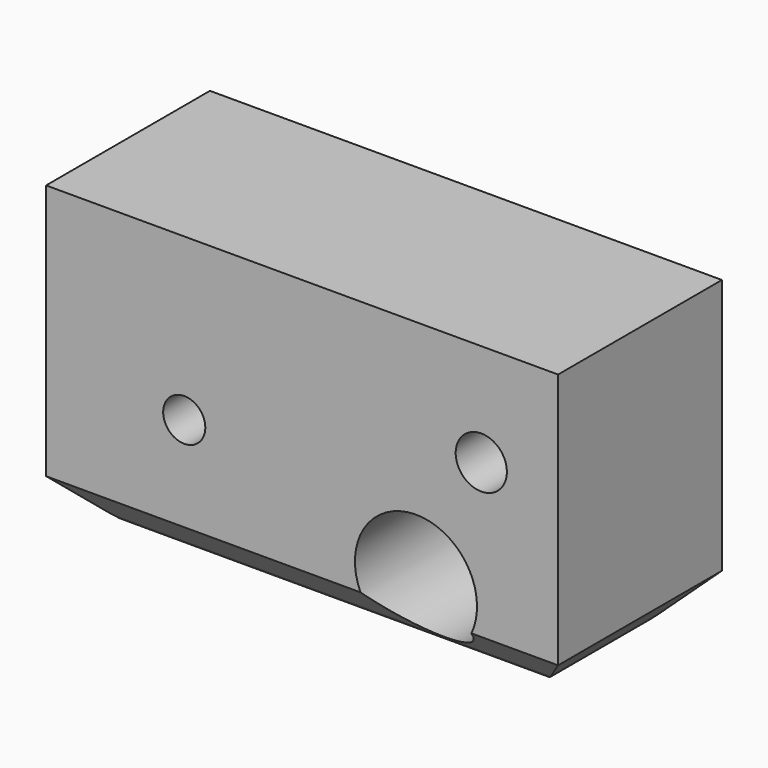
from build123d import *

# Parameters (mm, degrees)
F0_W        = 127
F0_H        = 76.2
F0_R        = 5.2244265331
F0_R_2      = 6.35
F1_DEPTH    = 50.8
F2_R        = 15.1393609574
F3_DEPTH    = 138.938
F4_T1_DEPTH = 116.1207478943
F4_T3_DEPTH = 192.3207478943
F5_R        = 12.7


# Not quite as in the source:
# - a fillet or chamfer that OpenCascade refuses, or shapes differently, is made with other operations: its cross-section is extruded or revolved along the edge and cut away or added


with BuildPart() as f1:
    # F0 (on Front) → F1 (new body)
    with BuildSketch(Plane.XZ):
        with Locations((-1.653669402, -66.8124542732)):
            Rectangle(F0_W, F0_H)
        with Locations((-30.8793820441, -68.7773153186)):
            Circle(F0_R, mode=Mode.SUBTRACT)
        with Locations((42.796330598, -54.1124542732)):
            Circle(F0_R_2, mode=Mode.SUBTRACT)
    extrude(amount=F1_DEPTH)

    # F2 (on face) → F3 (cut)
    with BuildSketch(Plane.XZ.offset(50.8)):
        with Locations((26.5990737826, -85.8985558152)):
            Circle(F2_R)
    extrude(amount=-F3_DEPTH, mode=Mode.SUBTRACT)

    # F4: chamfer of 12.7 on 4 edges, made by hand

    # F4_s2 → F4_t1 (cut)
    with BuildSketch(Plane.XZ.offset(-32.6603739472)):
        Polygon((61.846330598, -92.2124542732), (49.146330598, -104.9124542732), (61.846330598, -104.9124542732), align=None)
        Polygon((-65.153669402, -92.2124542732), (-52.453669402, -104.9124542732), (-65.153669402, -104.9124542732), align=None)
    extrude(amount=F4_T1_DEPTH, mode=Mode.SUBTRACT)

    # F4_s4 → F4_t3 (cut)
    with BuildSketch(Plane.YZ.offset(-97.8140433492)):
        Polygon((-50.8, -92.2124542732), (-38.1, -104.9124542732), (-50.8, -104.9124542732), align=None)
        Polygon((0, -92.2124542732), (-12.7, -104.9124542732), (0, -104.9124542732), align=None)
    extrude(amount=F4_T3_DEPTH, mode=Mode.SUBTRACT)

    # F5
    f5_edges = [f1.edges().sort_by_distance(p)[0] for p in [
        (-1.653669, -38.1, -104.912454),
        (-1.653669, -12.7, -104.912454),
        (49.146331, -25.4, -104.912454),
        (-52.453669, -25.4, -104.912454),
    ]]
    fillet(f5_edges, radius=F5_R)


solid = f1.part
